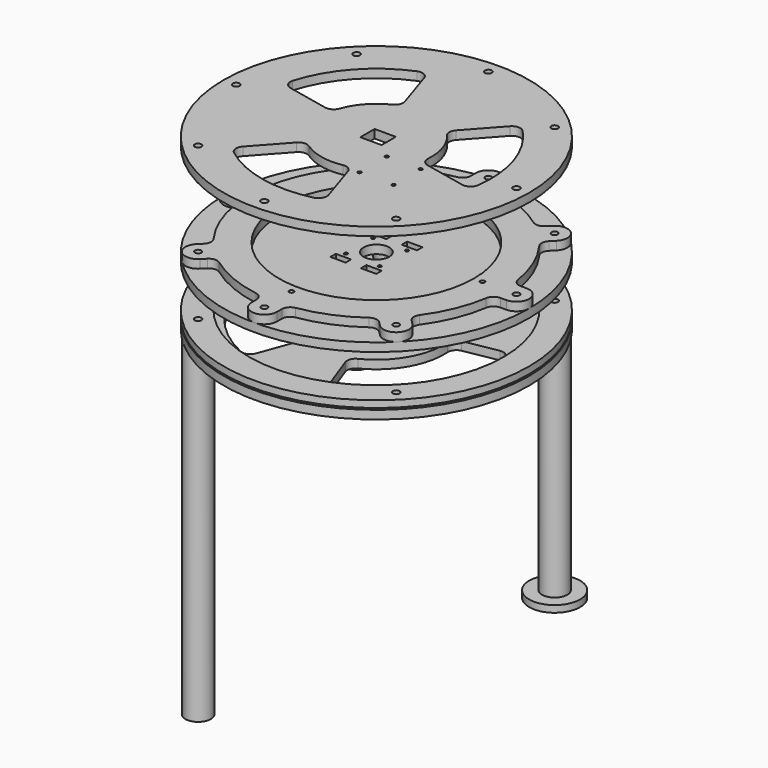
from build123d import *

# Parameters (mm, degrees)
F0_R      = 90
F0_R_2    = 2
F0_R_3    = 75
F1_DEPTH  = 4
F3_R      = 90
F3_R_2    = 2
F3_R_3    = 7.55
F4_DEPTH  = 5
F5_R      = 1
F6_DEPTH  = 5
F7_R      = 7.5
F8_DEPTH  = 195
F11_W     = 9
F11_H     = 4
F12_DEPTH = 5
F13_R     = 2
F13_R_2   = 1.85
F14_DEPTH = 5
F15_R     = 1.85
F15_R_2   = 1.35
F15_R_3   = 57.5
F16_DEPTH = 5
F17_R     = 5
F18_R     = 7.5
F18_R_2   = 2
F19_DEPTH = 140
F20_R     = 15
F20_R_2   = 7.5
F21_DEPTH = 4
F22_DEPTH = 2
F25_R     = 90
F25_R_2   = 2
F25_R_3   = 1
F26_DEPTH = 5
F27_DEPTH = 5
F28_R     = 7.5
F28_R_2   = 2
F29_DEPTH = 60
F30_R     = 2
F30_W     = 9
F30_H     = 4
F30_R_2   = 6.25
F31_DEPTH = 5
F33_DEPTH = 5


# Not quite as in the source:
# - a feature names something its author has since deleted; it is built from what else it names


with BuildPart() as f1:
    # F0 (on Top) → F1 (new body)
    with BuildSketch(Plane.XY):
        Circle(F0_R)
        with Locations((-58.3363094479, -58.3363094479)):
            Circle(F0_R_2, mode=Mode.SUBTRACT)
        with Locations((58.3363094479, -58.3363094479)):
            Circle(F0_R_2, mode=Mode.SUBTRACT)
        with Locations((-58.3363094479, 58.3363094479)):
            Circle(F0_R_2, mode=Mode.SUBTRACT)
        Circle(F0_R_3, mode=Mode.SUBTRACT)
        with Locations((58.3363094479, 58.3363094479)):
            Circle(F0_R_2, mode=Mode.SUBTRACT)
    extrude(amount=F1_DEPTH)


with BuildPart() as f4:
    # F3 (on offset) → F4 (new body)
    with BuildSketch(Plane(origin=(0, 0, -1), x_dir=(1, 0, 0), z_dir=(0, 0, -1))):
        Circle(F3_R)
        with Locations((-58.3363094479, -58.3363094479)):
            Circle(F3_R_2, mode=Mode.SUBTRACT)
        with Locations((58.3363094479, -58.3363094479)):
            Circle(F3_R_2, mode=Mode.SUBTRACT)
        with Locations((-58.3363094479, 58.3363094479)):
            Circle(F3_R_2, mode=Mode.SUBTRACT)
        Circle(F3_R_3, mode=Mode.SUBTRACT)
        with Locations((58.3363094479, 58.3363094479)):
            Circle(F3_R_2, mode=Mode.SUBTRACT)
    extrude(amount=F4_DEPTH)

    # F5 (on face) → F6 (cut, through all)
    with BuildSketch(Plane.XY.offset(-1)):
        with Locations((-10, 10)):
            Circle(F5_R)
        with Locations((10, 10)):
            Circle(F5_R)
        with Locations((-10, -10)):
            Circle(F5_R)
        with Locations((10, -10)):
            Circle(F5_R)
    extrude(amount=-F6_DEPTH, mode=Mode.SUBTRACT)


with BuildPart() as f8:
    # F7 (on face) → F8 (new body)
    with BuildSketch(Plane(origin=(0, 0, -6), x_dir=(1, 0, 0), z_dir=(0, 0, -1))):
        with Locations((-58.3363094479, 58.3363094479)):
            Circle(F7_R)
    extrude(amount=F8_DEPTH)


with BuildPart() as f10_1:
    # F10: instance of F4
    add(f4.part.mirror(Plane(origin=(0, 0, 14), x_dir=(1, 0, 0), z_dir=(0, 0, -1))))

    # F11 (on face) → F12 (cut, through all)
    with BuildSketch(Plane.XY.offset(34)):
        with Locations((9, -15)):
            Rectangle(F11_W, F11_H)
        with Locations((-9, -15)):
            Rectangle(F11_W, F11_H)
        with Locations((-9, 15)):
            Rectangle(F11_W, F11_H)
        with Locations((9, 15)):
            Rectangle(F11_W, F11_H)
    extrude(amount=-F12_DEPTH, mode=Mode.SUBTRACT)

    # F13 (on face) → F14 (join, through all)
    with BuildSketch(Plane.XY.offset(34)):
        with Locations((-58.3363094479, 58.3363094479)):
            Circle(F13_R)
        with Locations((-58.3363094479, 58.3363094479)):
            Circle(F13_R_2, mode=Mode.SUBTRACT)
        with Locations((-58.3363094479, -58.3363094479)):
            Circle(F13_R)
        with Locations((-58.3363094479, -58.3363094479)):
            Circle(F13_R_2, mode=Mode.SUBTRACT)
        with Locations((58.3363094479, -58.3363094479)):
            Circle(F13_R)
        with Locations((58.3363094479, -58.3363094479)):
            Circle(F13_R_2, mode=Mode.SUBTRACT)
        with Locations((58.3363094479, 58.3363094479)):
            Circle(F13_R)
        with Locations((58.3363094479, 58.3363094479)):
            Circle(F13_R_2, mode=Mode.SUBTRACT)
    extrude(amount=-F14_DEPTH)


with BuildPart() as f16:
    # F15 (on face) → F16 (new body)
    with BuildSketch(Plane.XY.offset(34)):
        with BuildLine():
            Line((58.0704781569, 47.4638764391), (63.6396103068, 53.033008589))
            ThreePointArc((63.6396103068, 53.033008589), (63.6396103068, 63.6396103068), (53.033008589, 63.6396103068))
            Line((53.033008589, 63.6396103068), (47.4638764391, 58.0704781569))
            ThreePointArc((47.4638764391, 58.0704781569), (28.7012574274, 69.2909649383), (7.5, 74.624057783))
            ThreePointArc((7.5, 74.624057783), (0, 75), (-7.5, 74.624057783))
            ThreePointArc((-7.5, 74.624057783), (-28.7012574274, 69.2909649383), (-47.4638764391, 58.0704781569))
            Line((-47.4638764391, 58.0704781569), (-53.033008589, 63.6396103068))
            ThreePointArc((-53.033008589, 63.6396103068), (-63.6396103068, 63.6396103068), (-63.6396103068, 53.033008589))
            Line((-63.6396103068, 53.033008589), (-58.0704781569, 47.4638764391))
            ThreePointArc((-58.0704781569, 47.4638764391), (-69.2909649383, 28.7012574274), (-74.624057783, 7.5))
            ThreePointArc((-74.624057783, 7.5), (-75, 0), (-74.624057783, -7.5))
            ThreePointArc((-74.624057783, -7.5), (-69.2909649383, -28.7012574274), (-58.0704781569, -47.4638764391))
            Line((-58.0704781569, -47.4638764391), (-63.6396103068, -53.033008589))
            ThreePointArc((-63.6396103068, -53.033008589), (-63.6396103068, -63.6396103068), (-53.033008589, -63.6396103068))
            Line((-53.033008589, -63.6396103068), (-47.4638764391, -58.0704781569))
            ThreePointArc((-47.4638764391, -58.0704781569), (-28.7012574274, -69.2909649383), (-7.5, -74.624057783))
            ThreePointArc((-7.5, -74.624057783), (0, -75), (7.5, -74.624057783))
            ThreePointArc((7.5, -74.624057783), (28.7012574274, -69.2909649383), (47.4638764391, -58.0704781569))
            Line((47.4638764391, -58.0704781569), (53.033008589, -63.6396103068))
            ThreePointArc((53.033008589, -63.6396103068), (63.6396103068, -63.6396103068), (63.6396103068, -53.033008589))
            Line((63.6396103068, -53.033008589), (58.0704781569, -47.4638764391))
            ThreePointArc((58.0704781569, -47.4638764391), (69.2909649383, -28.7012574274), (74.624057783, -7.5))
            ThreePointArc((74.624057783, -7.5), (75, 0), (74.624057783, 7.5))
            ThreePointArc((74.624057783, 7.5), (69.2909649383, 28.7012574274), (58.0704781569, 47.4638764391))
        make_face()
        with Locations((-58.3363094479, -58.3363094479)):
            Circle(F15_R, mode=Mode.SUBTRACT)
        with Locations((0, -62.5)):
            Circle(F15_R_2, mode=Mode.SUBTRACT)
        with Locations((58.3363094479, -58.3363094479)):
            Circle(F15_R, mode=Mode.SUBTRACT)
        with Locations((-62.5, 0)):
            Circle(F15_R_2, mode=Mode.SUBTRACT)
        with Locations((-58.3363094479, 58.3363094479)):
            Circle(F15_R, mode=Mode.SUBTRACT)
        Circle(F15_R_3, mode=Mode.SUBTRACT)
        with Locations((62.5, 0)):
            Circle(F15_R_2, mode=Mode.SUBTRACT)
        with Locations((0, 62.5)):
            Circle(F15_R_2, mode=Mode.SUBTRACT)
        with Locations((58.3363094479, 58.3363094479)):
            Circle(F15_R, mode=Mode.SUBTRACT)
        with BuildLine():
            Line((82.5, 7.5), (74.624057783, 7.5))
            ThreePointArc((74.624057783, 7.5), (75, 0), (74.624057783, -7.5))
            Line((74.624057783, -7.5), (82.5, -7.5))
            ThreePointArc((82.5, -7.5), (90, 0), (82.5, 7.5))
        make_face()
        with Locations((82.5, 0)):
            Circle(F15_R, mode=Mode.SUBTRACT)
        with BuildLine():
            ThreePointArc((-7.5, 74.624057783), (0, 75), (7.5, 74.624057783))
            Line((7.5, 74.624057783), (7.5, 82.5))
            ThreePointArc((7.5, 82.5), (0, 90), (-7.5, 82.5))
            Line((-7.5, 82.5), (-7.5, 74.624057783))
        make_face()
        with Locations((0, 82.5)):
            Circle(F15_R, mode=Mode.SUBTRACT)
        with BuildLine():
            Line((7.5, -82.5), (7.5, -74.624057783))
            ThreePointArc((7.5, -74.624057783), (0, -75), (-7.5, -74.624057783))
            Line((-7.5, -74.624057783), (-7.5, -82.5))
            ThreePointArc((-7.5, -82.5), (0, -90), (7.5, -82.5))
        make_face()
        with Locations((0, -82.5)):
            Circle(F15_R, mode=Mode.SUBTRACT)
        with BuildLine():
            ThreePointArc((-74.624057783, -7.5), (-75, 0), (-74.624057783, 7.5))
            Line((-74.624057783, 7.5), (-82.5, 7.5))
            ThreePointArc((-82.5, 7.5), (-90, 0), (-82.5, -7.5))
            Line((-82.5, -7.5), (-74.624057783, -7.5))
        make_face()
        with Locations((-82.5, 0)):
            Circle(F15_R, mode=Mode.SUBTRACT)
    extrude(amount=F16_DEPTH)

    # F17
    f17_edges = [f16.edges().sort_by_distance(p)[0] for p in [
        (-47.463876, 58.070478, 36.5),
        (47.463876, 58.070478, 36.5),
        (58.070478, 47.463876, 36.5),
        (58.070478, -47.463876, 36.5),
        (47.463876, -58.070478, 36.5),
        (-47.463876, -58.070478, 36.5),
        (-58.070478, -47.463876, 36.5),
        (-58.070478, 47.463876, 36.5),
        (74.624058, -7.5, 36.5),
        (74.624058, 7.5, 36.5),
        (7.5, 74.624058, 36.5),
        (-7.5, 74.624058, 36.5),
        (-74.624058, 7.5, 36.5),
        (-74.624058, -7.5, 36.5),
        (-7.5, -74.624058, 36.5),
        (7.5, -74.624058, 36.5),
    ]]
    fillet(f17_edges, radius=F17_R)


with BuildPart() as f19:
    # F18 (on face) → F19 (new body)
    with BuildSketch(Plane(origin=(0, 0, -6), x_dir=(1, 0, 0), z_dir=(0, 0, -1))):
        with Locations((58.3363094479, -58.3363094479)):
            Circle(F18_R)
        with Locations((58.3363094479, -58.3363094479)):
            Circle(F18_R_2, mode=Mode.SUBTRACT)
    extrude(amount=F19_DEPTH)


with BuildPart() as f21:
    # F20 (on face) → F21 (new body)
    with BuildSketch(Plane(origin=(0, 0, -146), x_dir=(1, 0, 0), z_dir=(0, 0, -1))):
        with Locations((58.3363094479, -58.3363094479)):
            Circle(F20_R)
        with Locations((58.3363094479, -58.3363094479)):
            Circle(F20_R_2, mode=Mode.SUBTRACT)
    extrude(amount=F21_DEPTH)

    # F22 (add): a face of the model
    f22_faces = [f19.part.faces().sort_by_distance(p)[0] for p in [
        (51.0484414822, 58.3363094479, -146),
    ]]
    extrude(f22_faces, amount=F22_DEPTH)


with BuildPart() as f24_1:
    # F24: instance of F4
    add(f4.part.mirror(Plane.XY.offset(44)))

    # F25 (on face) → F26 (join)
    with BuildSketch(Plane.XY.offset(94)):
        Circle(F25_R)
        with Locations((-58.3363094479, -58.3363094479)):
            Circle(F25_R_2, mode=Mode.SUBTRACT)
        with Locations((-10, -10)):
            Circle(F25_R_3, mode=Mode.SUBTRACT)
        with Locations((0, -82.5)):
            Circle(F25_R_2, mode=Mode.SUBTRACT)
        with Locations((58.3363094479, -58.3363094479)):
            Circle(F25_R_2, mode=Mode.SUBTRACT)
        with Locations((16.3, -32.75)):
            Circle(F25_R_3, mode=Mode.SUBTRACT)
        with Locations((36.3, -32.75)):
            Circle(F25_R_3, mode=Mode.SUBTRACT)
        with Locations((16.3, -12.75)):
            Circle(F25_R_3, mode=Mode.SUBTRACT)
        with Locations((10, -10)):
            Circle(F25_R_3, mode=Mode.SUBTRACT)
        with Locations((36.3, -12.75)):
            Circle(F25_R_3, mode=Mode.SUBTRACT)
        with Locations((-82.5, 0)):
            Circle(F25_R_2, mode=Mode.SUBTRACT)
        with Locations((-10, 10)):
            Circle(F25_R_3, mode=Mode.SUBTRACT)
        with Locations((-58.3363094479, 58.3363094479)):
            Circle(F25_R_2, mode=Mode.SUBTRACT)
        with BuildLine():
            ThreePointArc((5.4258639865, -5.25), (-7.55, 0), (5.4258639865, 5.25))
            Line((5.4258639865, 5.25), (7.25, 5.25))
            Line((7.25, 5.25), (7.25, 2.1071307506))
            ThreePointArc((7.25, 2.1071307506), (7.4746237363, 1.0641898327), (7.55, 0))
            ThreePointArc((7.55, 0), (7.4746237363, -1.0641898327), (7.25, -2.1071307506))
            Line((7.25, -2.1071307506), (7.25, -5.25))
            Line((7.25, -5.25), (5.4258639865, -5.25))
        make_face(mode=Mode.SUBTRACT)
        with Locations((10, 10)):
            Circle(F25_R_3, mode=Mode.SUBTRACT)
        with Locations((82.5, 0)):
            Circle(F25_R_2, mode=Mode.SUBTRACT)
        with Locations((0, 82.5)):
            Circle(F25_R_2, mode=Mode.SUBTRACT)
        with Locations((58.3363094479, 58.3363094479)):
            Circle(F25_R_2, mode=Mode.SUBTRACT)
        with BuildLine():
            Line((-5.25, -5.25), (-5.25, 5.25))
            Line((-5.25, 5.25), (5.4258639865, 5.25))
            ThreePointArc((5.4258639865, 5.25), (-7.55, 0), (5.4258639865, -5.25))
            Line((5.4258639865, -5.25), (-5.25, -5.25))
        make_face()
        with Locations((-10, -10)):
            Circle(F25_R_3)
        with Locations((-10, 10)):
            Circle(F25_R_3)
        with Locations((10, 10)):
            Circle(F25_R_3)
        with Locations((10, -10)):
            Circle(F25_R_3)
        with BuildLine():
            ThreePointArc((7.55, 0), (7.4746237363, 1.0641898327), (7.25, 2.1071307506))
            Line((7.25, 2.1071307506), (7.25, -2.1071307506))
            ThreePointArc((7.25, -2.1071307506), (7.4746237363, -1.0641898327), (7.55, 0))
        make_face()
    extrude(amount=-F26_DEPTH)

    # F25 (on face) → F27 (cut)
    with BuildSketch(Plane.XY.offset(94)):
        with Locations((0, -82.5)):
            Circle(F25_R_2)
        with Locations((82.5, 0)):
            Circle(F25_R_2)
        with Locations((0, 82.5)):
            Circle(F25_R_2)
        with Locations((-82.5, 0)):
            Circle(F25_R_2)
        with BuildLine():
            Line((7.25, 5.25), (5.4258639865, 5.25))
            ThreePointArc((5.4258639865, 5.25), (6.5298383388, 3.7899487159), (7.25, 2.1071307506))
            Line((7.25, 2.1071307506), (7.25, 5.25))
        make_face()
        with BuildLine():
            ThreePointArc((7.25, -2.1071307506), (6.5298383388, -3.7899487159), (5.4258639865, -5.25))
            Line((5.4258639865, -5.25), (7.25, -5.25))
            Line((7.25, -5.25), (7.25, -2.1071307506))
        make_face()
        with Locations((16.3, -12.75)):
            Circle(F25_R_3)
        with Locations((36.3, -12.75)):
            Circle(F25_R_3)
        with Locations((36.3, -32.75)):
            Circle(F25_R_3)
        with Locations((16.3, -32.75)):
            Circle(F25_R_3)
    extrude(amount=-F27_DEPTH, mode=Mode.SUBTRACT)

    # F32 (on face) → F33 (cut, through all)
    with BuildSketch(Plane.XY.offset(94)):
        with BuildLine():
            ThreePointArc((-41.6866219664, -46.2976840569), (-42.9495673901, -50.1046932427), (-41.0085696662, -53.6148040557))
            ThreePointArc((-41.0085696662, -53.6148040557), (-14.0340391302, -66.0249630495), (15.6560871221, -65.6592486709))
            ThreePointArc((15.6560871221, -65.6592486709), (18.8569674651, -63.2420777803), (19.2516595464, -59.2505156493))
            Line((19.2516595464, -59.2505156493), (11.4846697062, -35.3461788846))
            ThreePointArc((11.4846697062, -35.3461788846), (9.2919343632, -32.5978559268), (5.8321355081, -31.9724286756))
            ThreePointArc((5.8321355081, -31.9724286756), (-6.7571299516, -31.7897970238), (-18.3322792122, -26.8361237679))
            ThreePointArc((-18.3322792122, -26.8361237679), (-21.7473469213, -26.0002530202), (-24.8683539877, -27.6191051619))
            Line((-24.8683539877, -27.6191051619), (-41.6866219664, -46.2976840569))
        make_face()
        with BuildLine():
            Line((-60.9382815128, 12.9528315924), (-36.3530236938, 7.7270737227))
            ThreePointArc((-36.3530236938, 7.7270737227), (-32.8765385231, 8.2518767546), (-30.6050032078, 10.9354368295))
            ThreePointArc((-30.6050032078, 10.9354368295), (-24.152206828, 21.7467447067), (-14.074625316, 29.294281391))
            ThreePointArc((-14.074625316, 29.294281391), (-11.6432061597, 31.8338814089), (-11.4846697062, 35.3461788846))
            Line((-11.4846697062, 35.3461788846), (-19.2516595464, 59.2505156493))
            ThreePointArc((-19.2516595464, 59.2505156493), (-21.9171535019, 62.2477630628), (-25.9274974981, 62.3218651316))
            ThreePointArc((-25.9274974981, 62.3218651316), (-50.1622757197, 45.1663159292), (-64.6906209034, 19.2710551638))
            ThreePointArc((-64.6906209034, 19.2710551638), (-64.1977296784, 15.290426027), (-60.9382815128, 12.9528315924))
        make_face()
        with BuildLine():
            ThreePointArc((32.4069045282, -2.4581576231), (33.390553081, -5.8336283887), (36.3530236938, -7.7270737227))
            Line((36.3530236938, -7.7270737227), (60.9382815128, -12.9528315924))
            ThreePointArc((60.9382815128, -12.9528315924), (64.8667208921, -12.1430698201), (66.9360671643, -8.7070610759))
            ThreePointArc((66.9360671643, -8.7070610759), (64.1963148499, 20.8586471203), (49.0345337813, 46.3881935071))
            ThreePointArc((49.0345337813, 46.3881935071), (45.3407622133, 47.9516517532), (41.6866219664, 46.2976840569))
            Line((41.6866219664, 46.2976840569), (24.8683539877, 27.6191051619))
            ThreePointArc((24.8683539877, 27.6191051619), (23.5846041599, 24.3459791722), (24.7728676997, 21.0369918461))
            ThreePointArc((24.7728676997, 21.0369918461), (30.9093367796, 10.0430523172), (32.4069045282, -2.4581576231))
        make_face()
    extrude(amount=-F33_DEPTH, mode=Mode.SUBTRACT)


with BuildPart() as f29:
    # F28 (on face) → F29 (new body)
    with BuildSketch(Plane(origin=(0, 0, -6), x_dir=(1, 0, 0), z_dir=(0, 0, -1))):
        with Locations((-58.3363094479, -58.3363094479)):
            Circle(F28_R)
        with Locations((-58.3363094479, -58.3363094479)):
            Circle(F28_R_2, mode=Mode.SUBTRACT)
    extrude(amount=F29_DEPTH)


with BuildPart() as f4_1:
    add(f4.part)

    # F30 (on face) → F31 (cut)
    with BuildSketch(Plane(origin=(0, 0, -6), x_dir=(1, 0, 0), z_dir=(0, 0, -1))):
        with BuildLine():
            ThreePointArc((-22.1654386253, 60.8990421152), (-24.9267954635, 63.7984553985), (-28.9303557084, 63.7419368908))
            ThreePointArc((-28.9303557084, 63.7419368908), (-60.6217782649, 35), (-69.667314488, -6.8165454614))
            ThreePointArc((-69.667314488, -6.8165454614), (-67.7144808291, -10.3119895929), (-63.8228368505, -11.2536881221))
            Line((-63.8228368505, -11.2536881221), (-44.0419416101, -7.7657825886))
            ThreePointArc((-44.0419416101, -7.7657825886), (-40.9803414393, -5.9330783655), (-39.9201622208, -2.5259945099))
            ThreePointArc((-39.9201622208, -2.5259945099), (-34.6410161514, 20), (-17.7725056951, 35.8348718613))
            ThreePointArc((-17.7725056951, 35.8348718613), (-15.3519741325, 38.456555925), (-15.295605803, 42.0243315606))
            Line((-15.295605803, 42.0243315606), (-22.1654386253, 60.8990421152))
        make_face()
        with BuildLine():
            ThreePointArc((28.9303557084, 63.7419368908), (24.9267954635, 63.7984553985), (22.1654386253, 60.8990421152))
            Line((22.1654386253, 60.8990421152), (15.295605803, 42.0243315606))
            ThreePointArc((15.295605803, 42.0243315606), (15.3519741325, 38.456555925), (17.7725056951, 35.8348718613))
            ThreePointArc((17.7725056951, 35.8348718613), (34.6410161514, 20), (39.9201622208, -2.5259945099))
            ThreePointArc((39.9201622208, -2.5259945099), (40.9803414393, -5.9330783655), (44.0419416101, -7.7657825886))
            Line((44.0419416101, -7.7657825886), (63.8228368505, -11.2536881221))
            ThreePointArc((63.8228368505, -11.2536881221), (67.7144808291, -10.3119895929), (69.667314488, -6.8165454614))
            ThreePointArc((69.667314488, -6.8165454614), (60.6217782649, 35), (28.9303557084, 63.7419368908))
        make_face()
        with BuildLine():
            Line((-28.7463358071, -34.258548972), (-41.6573982253, -49.6453539931))
            ThreePointArc((-41.6573982253, -49.6453539931), (-42.7876853656, -53.4864658056), (-40.7369587797, -56.9253914293))
            ThreePointArc((-40.7369587797, -56.9253914293), (0, -70), (40.7369587797, -56.9253914293))
            ThreePointArc((40.7369587797, -56.9253914293), (42.7876853656, -53.4864658056), (41.6573982253, -49.6453539931))
            Line((41.6573982253, -49.6453539931), (28.7463358071, -34.258548972))
            ThreePointArc((28.7463358071, -34.258548972), (25.6283673069, -32.5234775594), (22.1476565258, -33.3088773515))
            ThreePointArc((22.1476565258, -33.3088773515), (0, -40), (-22.1476565258, -33.3088773515))
            ThreePointArc((-22.1476565258, -33.3088773515), (-25.6283673069, -32.5234775594), (-28.7463358071, -34.258548972))
        make_face()
        with Locations((58.3363094479, 58.3363094479)):
            Circle(F30_R)
        with Locations((0, 82.5)):
            Circle(F30_R)
        with Locations((-58.3363094479, 58.3363094479)):
            Circle(F30_R)
        with Locations((-82.5, 0)):
            Circle(F30_R)
        with Locations((-58.3363094479, -58.3363094479)):
            Circle(F30_R)
        with Locations((0, -82.5)):
            Circle(F30_R)
        with Locations((58.3363094479, -58.3363094479)):
            Circle(F30_R)
        with Locations((82.5, 0)):
            Circle(F30_R)
        with Locations((-9, 15)):
            Rectangle(F30_W, F30_H)
        with Locations((-9, -15)):
            Rectangle(F30_W, F30_H)
        with Locations((9, -15)):
            Rectangle(F30_W, F30_H)
        with Locations((9, 15)):
            Rectangle(F30_W, F30_H)
        with Locations((0, 27.35)):
            Circle(F30_R_2)
    extrude(amount=-F31_DEPTH, mode=Mode.SUBTRACT)


solid = Compound([f1.part, f8.part, f10_1.part, f16.part, f19.part, f21.part, f24_1.part, f29.part, f4_1.part])
